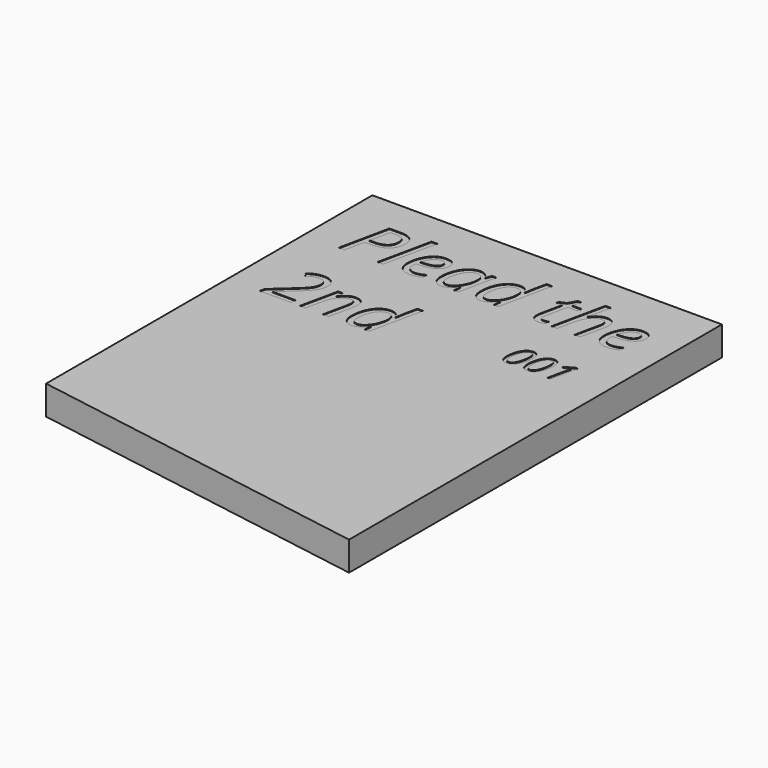
from build123d import *

# Parameters (mm, degrees)
F1_DEPTH     = 3.175
F2_TEXT_SIZE = 7.6612751197
F3_DEPTH     = 0.0762
F4_TEXT_SIZE = 4.1584748565
F5_DEPTH     = 0.0762


# Not quite as in the source:
# - Text() gives the source's letters only with a copy of the font that has no kerning and outlines rounded to 1/6400 em; it was checked with that copy


with BuildPart() as f1:
    # F0 (on Top) → F1 (new body)
    with BuildSketch(Plane.XY):
        Polygon((19.05, 25.4), (-19.05, 25.4), (-19.05, -19.05), (19.05, -25.4), align=None)
    extrude(amount=F1_DEPTH)

    # F2 (on face) → F3 (cut)
    with BuildSketch(Plane.XY.offset(3.175)):
        with Locations((-15.5723319007, 16.0623274433)):
            Text('Plead the', F2_TEXT_SIZE, font='Open Sans', font_style=FontStyle.ITALIC, text_align=(TextAlign.LEFT, TextAlign.BOTTOM))
        with Locations((-15.5723319007, 5.6429932805)):
            Text('2nd', F2_TEXT_SIZE, font='Open Sans', font_style=FontStyle.ITALIC, text_align=(TextAlign.LEFT, TextAlign.BOTTOM))
    extrude(amount=-F3_DEPTH, mode=Mode.SUBTRACT)

    # F4 (on face) → F5 (cut)
    with BuildSketch(Plane.XY.offset(3.175)):
        with Locations((8.1659227498, 8.4220085949)):
            Text('001', F4_TEXT_SIZE, font='Open Sans', font_style=FontStyle.ITALIC, text_align=(TextAlign.LEFT, TextAlign.BOTTOM))
    extrude(amount=-F5_DEPTH, mode=Mode.SUBTRACT)


solid = f1.part
